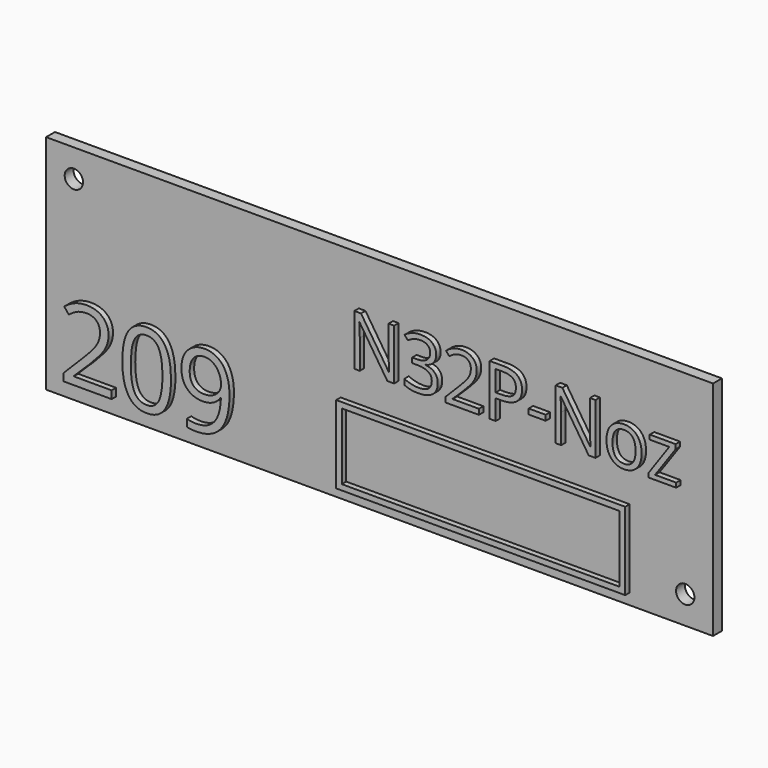
from build123d import *

# Parameters (mm, degrees)
F0_W         = 120
F0_H         = 40
F1_DEPTH     = 2
F3_D         = 3.3
F4_TEXT_SIZE = 12.8419503712
F5_DEPTH     = 1
F6_TEXT_SIZE = 18.5356140827
F7_DEPTH     = 1
F8_W         = 52
F8_H         = 14
F8_W_2       = 49.99999962
F8_H_2       = 11.99999962
F9_DEPTH     = 1


# Not quite as in the source:
# - Text() gives the source's letters only with a copy of the font that has no kerning and outlines rounded to 1/6400 em; it was checked with that copy


with BuildPart() as f1:
    # F0 (on Front) → F1 (new body)
    with BuildSketch(Plane.XZ):
        Rectangle(F0_W, F0_H)
    extrude(amount=F1_DEPTH)

    # F3 (through all)
    with Locations(Plane.XZ.offset(2)):
        with Locations((-55, 15), (55, -15)):
            Hole(F3_D / 2)

    # F4 (on face) → F5 (join)
    with BuildSketch(Plane.XZ.offset(2)):
        with Locations((-5, 2)):
            Text('N32P-Noz', F4_TEXT_SIZE, font='Open Sans', text_align=(TextAlign.LEFT, TextAlign.BOTTOM))
    extrude(amount=F5_DEPTH)

    # F6 (on face) → F7 (join)
    with BuildSketch(Plane.XZ.offset(2)):
        with Locations((-57, -17)):
            Text('209', F6_TEXT_SIZE, font='Open Sans', text_align=(TextAlign.LEFT, TextAlign.BOTTOM))
    extrude(amount=F7_DEPTH)

    # F8 (on face) → F9 (join)
    with BuildSketch(Plane.XZ.offset(2)):
        with Locations((19, -11)):
            Rectangle(F8_W, F8_H)
        with Locations((19, -11)):
            Rectangle(F8_W_2, F8_H_2, mode=Mode.SUBTRACT)
    extrude(amount=F9_DEPTH)


solid = f1.part
